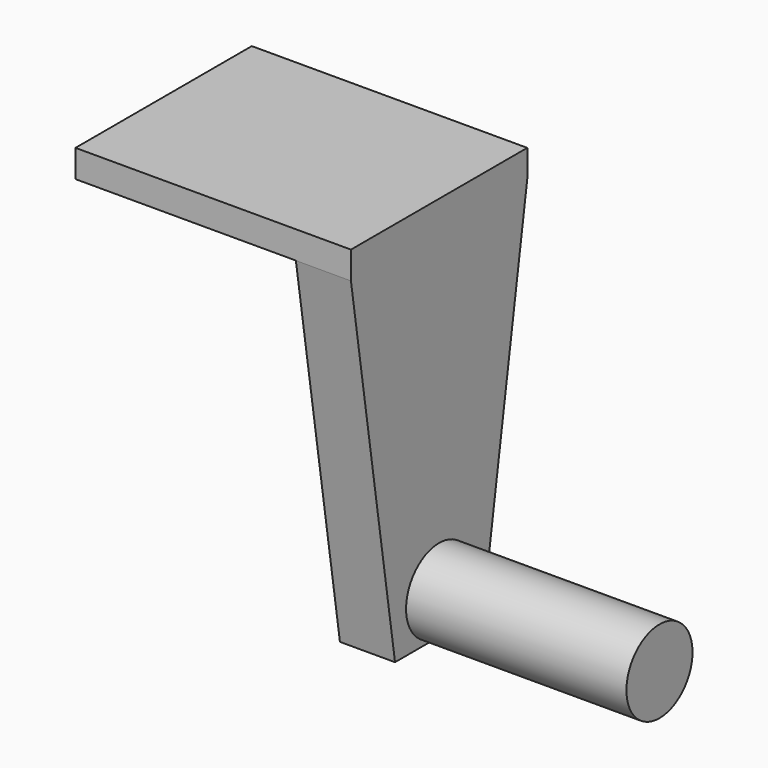
from build123d import *

# Parameters (mm, degrees)
F0_W     = 31.75
F0_H     = 25.4
F2_DEPTH = 3.175
F3_DEPTH = 6.35
F4_DEPTH = 25.4


# Not quite as in the source:
# - a length typed as a fraction of an inch, garbled in the dataset ("3 / 203.2 mm" for 3/8 in), is restored
# - a feature names something its author has since deleted; it is built from what else it names


with BuildPart() as f2:
    # F0 (on Top) → F2 (new body)
    with BuildSketch(Plane.XY):
        with Locations((-15.875, 0)):
            Rectangle(F0_W, F0_H)
    extrude(amount=F2_DEPTH)

    # F1 (on Right) → F3 (join)
    with BuildSketch(Plane.YZ):
        Polygon((12.7, 0), (-12.7, 0), (-6.35, -41.275), (0, -41.275), (6.35, -41.275), align=None)
        with BuildLine():
            ThreePointArc((4.7625, -36.5125), (3.3675960454, -39.8800960454), (0, -41.275))
            ThreePointArc((0, -41.275), (-3.3675960454, -33.1449039546), (4.7625, -36.5125))
        make_face(mode=Mode.SUBTRACT)
        with BuildLine():
            ThreePointArc((4.7625, -36.5125), (-3.3675960454, -33.1449039546), (0, -41.275))
            ThreePointArc((0, -41.275), (3.3675960454, -39.8800960454), (4.7625, -36.5125))
        make_face()
    extrude(amount=-F3_DEPTH)


with BuildPart() as f4:
    # F1 (on Right) → F4 (new body)
    with BuildSketch(Plane.YZ):
        with BuildLine():
            ThreePointArc((4.7625, -36.5125), (-3.3675960454, -33.1449039546), (0, -41.275))
            ThreePointArc((0, -41.275), (3.3675960454, -39.8800960454), (4.7625, -36.5125))
        make_face()
    extrude(amount=F4_DEPTH)


solid = Compound([f2.part, f4.part])
